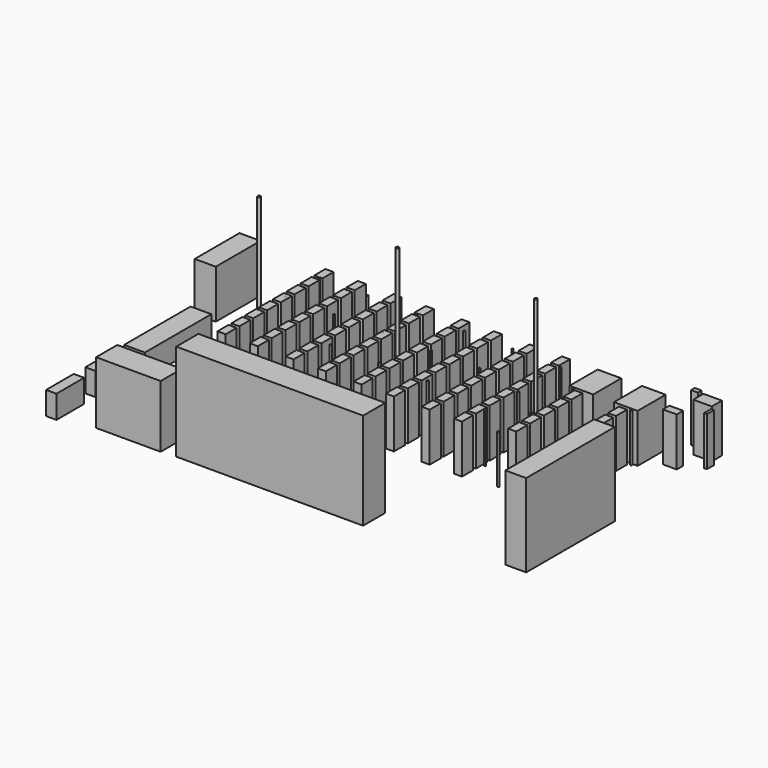
from build123d import *

# Parameters (mm, degrees)
F1_R      = 63.5
F12_DEPTH = 5486.4
F7_W      = 1041.4
F7_H      = 515.62
F13_DEPTH = 2133.6
F7_W_2    = 355.6
F7_H_2    = 609.6
F8_W      = 355.6
F8_H      = 609.6
F14_DEPTH = 2133.6
F9_W      = 355.6
F9_H      = 609.6
F15_DEPTH = 2133.6
F10_W     = 355.6
F10_H     = 609.6
F16_DEPTH = 2133.6
F11_W     = 355.6
F11_H     = 609.6
F17_DEPTH = 2133.6
F6_W      = 914.4
F6_H      = 4876.8
F18_DEPTH = 3657.6
F5_W      = 8229.6
F5_H      = 1219.2
F19_DEPTH = 4267.2
F4_W      = 1422.4
F4_H      = 1168.4
F20_DEPTH = 2743.2
F3_W      = 914.4
F3_H      = 1828.8
F21_DEPTH = 1016
F3_W_2    = 457.2
F3_H_2    = 1524
F3_H_3    = 1219.2
F2_W      = 812.8
F2_H      = 558.8
F22_DEPTH = 2133.6
F2_W_2    = 609.6
F2_H_2    = 355.6
F2_W_3    = 304.8
F2_H_3    = 203.2
F2_W_4    = 127
F2_H_4    = 406.4
F24_W     = 927.1
F24_H     = 1231.9
F25_DEPTH = 2133.6
F24_R     = 38.1


# Not quite as in the source:
# - the program builds the solid bodies; features that only make, move or delete a surface that nothing else refers to are left out


with BuildPart() as f12:
    # F1 (on face) → F12 (new body)
    with BuildSketch(Plane.XY):
        with Locations((-7657.7831685632, 0)):
            Circle(F1_R)
    extrude(amount=F12_DEPTH)


with BuildPart() as f12b:
    # F1 (on face) → F12, piece 2 (new body)
    with BuildSketch(Plane.XY):
        with Locations((-1561.7831685632, 0)):
            Circle(F1_R)
    extrude(amount=F12_DEPTH)


with BuildPart() as f12c:
    # F1 (on face) → F12, piece 3 (new body)
    with BuildSketch(Plane.XY):
        with Locations((4534.2168314368, 0)):
            Circle(F1_R)
    extrude(amount=F12_DEPTH)


with BuildPart() as f13:
    # F7 (on face) → F13 (new body)
    with BuildSketch(Plane.XY):
        with Locations((7941.9141265869, 1461.77)):
            Rectangle(F7_W, F7_H)
        with Locations((7941.9141265869, 1977.39)):
            Rectangle(F7_W, F7_H)
        with Locations((7941.9141265869, 946.15)):
            Rectangle(F7_W, F7_H)
    extrude(amount=F13_DEPTH)


with BuildPart() as f13b:
    # F7 (on face) → F13, piece 2 (new body)
    with BuildSketch(Plane.XY):
        with Locations((5986.1141265869, 1461.77)):
            Rectangle(F7_W, F7_H)
        with Locations((5986.1141265869, 1977.39)):
            Rectangle(F7_W, F7_H)
        with Locations((5986.1141265869, 946.15)):
            Rectangle(F7_W, F7_H)
    extrude(amount=F13_DEPTH)


with BuildPart() as f13c:
    # F7 (on face) → F13, piece 3 (new body)
    with BuildSketch(Plane.XY):
        with Locations((5986.1141265869, 231.14)):
            Rectangle(F7_W_2, F7_H_2)
    extrude(amount=F13_DEPTH)


with BuildPart() as f13d:
    # F7 (on face) → F13, piece 4 (new body)
    with BuildSketch(Plane.XY):
        with Locations((5986.1141265869, -530.86)):
            Rectangle(F7_W_2, F7_H_2)
    extrude(amount=F13_DEPTH)


with BuildPart() as f13e:
    # F7 (on face) → F13, piece 5 (new body)
    with BuildSketch(Plane.XY):
        with Locations((5986.1141265869, -1292.86)):
            Rectangle(F7_W_2, F7_H_2)
    extrude(amount=F13_DEPTH)


with BuildPart() as f13f:
    # F7 (on face) → F13, piece 6 (new body)
    with BuildSketch(Plane.XY):
        with Locations((7941.9141265869, 231.14)):
            Rectangle(F7_W_2, F7_H_2)
    extrude(amount=F13_DEPTH)


with BuildPart() as f13g:
    # F7 (on face) → F13, piece 7 (new body)
    with BuildSketch(Plane.XY):
        with Locations((7941.9141265869, -530.86)):
            Rectangle(F7_W_2, F7_H_2)
    extrude(amount=F13_DEPTH)


with BuildPart() as f13h:
    # F7 (on face) → F13, piece 8 (new body)
    with BuildSketch(Plane.XY):
        with Locations((7941.9141265869, -1292.86)):
            Rectangle(F7_W_2, F7_H_2)
    extrude(amount=F13_DEPTH)


with BuildPart() as f13i:
    # F7 (on face) → F13, piece 9 (new body)
    with BuildSketch(Plane.XY):
        with Locations((5986.1141265869, -2054.86)):
            Rectangle(F7_W_2, F7_H_2)
    extrude(amount=F13_DEPTH)


with BuildPart() as f13j:
    # F7 (on face) → F13, piece 10 (new body)
    with BuildSketch(Plane.XY):
        with Locations((7941.9141265869, -2054.86)):
            Rectangle(F7_W_2, F7_H_2)
    extrude(amount=F13_DEPTH)


with BuildPart() as f13k:
    # F7 (on face) → F13, piece 11 (new body)
    with BuildSketch(Plane.XY):
        with Locations((5986.1141265869, -2816.86)):
            Rectangle(F7_W_2, F7_H_2)
    extrude(amount=F13_DEPTH)


with BuildPart() as f13l:
    # F7 (on face) → F13, piece 12 (new body)
    with BuildSketch(Plane.XY):
        with Locations((7941.9141265869, -2816.86)):
            Rectangle(F7_W_2, F7_H_2)
    extrude(amount=F13_DEPTH)


with BuildPart() as f14:
    # F8 (on face) → F14 (new body)
    with BuildSketch(Plane.XY):
        with Locations((4068.4141265869, 1930.4)):
            Rectangle(F8_W, F8_H)
    extrude(amount=F14_DEPTH)


with BuildPart() as f14b:
    # F8 (on face) → F14, piece 2 (new body)
    with BuildSketch(Plane.XY):
        with Locations((4068.4141265869, 1168.4)):
            Rectangle(F8_W, F8_H)
    extrude(amount=F14_DEPTH)


with BuildPart() as f14c:
    # F8 (on face) → F14, piece 3 (new body)
    with BuildSketch(Plane.XY):
        with Locations((2646.0141265869, 1930.4)):
            Rectangle(F8_W, F8_H)
    extrude(amount=F14_DEPTH)


with BuildPart() as f14d:
    # F8 (on face) → F14, piece 4 (new body)
    with BuildSketch(Plane.XY):
        with Locations((2646.0141265869, 1168.4)):
            Rectangle(F8_W, F8_H)
    extrude(amount=F14_DEPTH)


with BuildPart() as f14e:
    # F8 (on face) → F14, piece 5 (new body)
    with BuildSketch(Plane.XY):
        with Locations((2646.0141265869, 406.4)):
            Rectangle(F8_W, F8_H)
    extrude(amount=F14_DEPTH)


with BuildPart() as f14f:
    # F8 (on face) → F14, piece 6 (new body)
    with BuildSketch(Plane.XY):
        with Locations((4068.4141265869, 406.4)):
            Rectangle(F8_W, F8_H)
    extrude(amount=F14_DEPTH)


with BuildPart() as f14g:
    # F8 (on face) → F14, piece 7 (new body)
    with BuildSketch(Plane.XY):
        with Locations((2646.0141265869, -355.6)):
            Rectangle(F8_W, F8_H)
    extrude(amount=F14_DEPTH)


with BuildPart() as f14h:
    # F8 (on face) → F14, piece 8 (new body)
    with BuildSketch(Plane.XY):
        with Locations((4068.4141265869, -355.6)):
            Rectangle(F8_W, F8_H)
    extrude(amount=F14_DEPTH)


with BuildPart() as f14i:
    # F8 (on face) → F14, piece 9 (new body)
    with BuildSketch(Plane.XY):
        with Locations((2646.0141265869, -1117.6)):
            Rectangle(F8_W, F8_H)
    extrude(amount=F14_DEPTH)


with BuildPart() as f14j:
    # F8 (on face) → F14, piece 10 (new body)
    with BuildSketch(Plane.XY):
        with Locations((4068.4141265869, -1117.6)):
            Rectangle(F8_W, F8_H)
    extrude(amount=F14_DEPTH)


with BuildPart() as f14k:
    # F8 (on face) → F14, piece 11 (new body)
    with BuildSketch(Plane.XY):
        with Locations((2646.0141265869, -1879.6)):
            Rectangle(F8_W, F8_H)
    extrude(amount=F14_DEPTH)


with BuildPart() as f14l:
    # F8 (on face) → F14, piece 12 (new body)
    with BuildSketch(Plane.XY):
        with Locations((4068.4141265869, -1879.6)):
            Rectangle(F8_W, F8_H)
    extrude(amount=F14_DEPTH)


with BuildPart() as f14m:
    # F8 (on face) → F14, piece 13 (new body)
    with BuildSketch(Plane.XY):
        with Locations((2646.014126587, -2641.6)):
            Rectangle(F8_W, F8_H)
    extrude(amount=F14_DEPTH)


with BuildPart() as f14n:
    # F8 (on face) → F14, piece 14 (new body)
    with BuildSketch(Plane.XY):
        with Locations((4068.4141265869, -2641.6)):
            Rectangle(F8_W, F8_H)
    extrude(amount=F14_DEPTH)


with BuildPart() as f14o:
    # F8 (on face) → F14, piece 15 (new body)
    with BuildSketch(Plane.XY):
        with Locations((2646.0141265869, -3403.6)):
            Rectangle(F8_W, F8_H)
    extrude(amount=F14_DEPTH)


with BuildPart() as f14p:
    # F8 (on face) → F14, piece 16 (new body)
    with BuildSketch(Plane.XY):
        with Locations((4068.4141265869, -3403.6)):
            Rectangle(F8_W, F8_H)
    extrude(amount=F14_DEPTH)


with BuildPart() as f15:
    # F9 (on face) → F15 (new body)
    with BuildSketch(Plane.XY):
        with Locations((1071.2141265869, 1930.4)):
            Rectangle(F9_W, F9_H)
    extrude(amount=F15_DEPTH)


with BuildPart() as f15b:
    # F9 (on face) → F15, piece 2 (new body)
    with BuildSketch(Plane.XY):
        with Locations((1071.2141265869, 1168.4)):
            Rectangle(F9_W, F9_H)
    extrude(amount=F15_DEPTH)


with BuildPart() as f15c:
    # F9 (on face) → F15, piece 3 (new body)
    with BuildSketch(Plane.XY):
        with Locations((-351.1858734131, 1930.4)):
            Rectangle(F9_W, F9_H)
    extrude(amount=F15_DEPTH)


with BuildPart() as f15d:
    # F9 (on face) → F15, piece 4 (new body)
    with BuildSketch(Plane.XY):
        with Locations((-351.1858734131, 1168.4)):
            Rectangle(F9_W, F9_H)
    extrude(amount=F15_DEPTH)


with BuildPart() as f15e:
    # F9 (on face) → F15, piece 5 (new body)
    with BuildSketch(Plane.XY):
        with Locations((-351.1858734131, 406.4)):
            Rectangle(F9_W, F9_H)
    extrude(amount=F15_DEPTH)


with BuildPart() as f15f:
    # F9 (on face) → F15, piece 6 (new body)
    with BuildSketch(Plane.XY):
        with Locations((1071.2141265869, 406.4)):
            Rectangle(F9_W, F9_H)
    extrude(amount=F15_DEPTH)


with BuildPart() as f15g:
    # F9 (on face) → F15, piece 7 (new body)
    with BuildSketch(Plane.XY):
        with Locations((-351.1858734131, -355.6)):
            Rectangle(F9_W, F9_H)
    extrude(amount=F15_DEPTH)


with BuildPart() as f15h:
    # F9 (on face) → F15, piece 8 (new body)
    with BuildSketch(Plane.XY):
        with Locations((1071.2141265869, -355.6)):
            Rectangle(F9_W, F9_H)
    extrude(amount=F15_DEPTH)


with BuildPart() as f15i:
    # F9 (on face) → F15, piece 9 (new body)
    with BuildSketch(Plane.XY):
        with Locations((-351.1858734131, -1117.6)):
            Rectangle(F9_W, F9_H)
    extrude(amount=F15_DEPTH)


with BuildPart() as f15j:
    # F9 (on face) → F15, piece 10 (new body)
    with BuildSketch(Plane.XY):
        with Locations((1071.2141265869, -1117.6)):
            Rectangle(F9_W, F9_H)
    extrude(amount=F15_DEPTH)


with BuildPart() as f15k:
    # F9 (on face) → F15, piece 11 (new body)
    with BuildSketch(Plane.XY):
        with Locations((-351.1858734131, -1879.6)):
            Rectangle(F9_W, F9_H)
    extrude(amount=F15_DEPTH)


with BuildPart() as f15l:
    # F9 (on face) → F15, piece 12 (new body)
    with BuildSketch(Plane.XY):
        with Locations((1071.2141265869, -1879.6)):
            Rectangle(F9_W, F9_H)
    extrude(amount=F15_DEPTH)


with BuildPart() as f15m:
    # F9 (on face) → F15, piece 13 (new body)
    with BuildSketch(Plane.XY):
        with Locations((-351.1858734131, -2641.6)):
            Rectangle(F9_W, F9_H)
    extrude(amount=F15_DEPTH)


with BuildPart() as f15n:
    # F9 (on face) → F15, piece 14 (new body)
    with BuildSketch(Plane.XY):
        with Locations((1071.2141265869, -2641.6)):
            Rectangle(F9_W, F9_H)
    extrude(amount=F15_DEPTH)


with BuildPart() as f15o:
    # F9 (on face) → F15, piece 15 (new body)
    with BuildSketch(Plane.XY):
        with Locations((-351.185873413, -3403.6)):
            Rectangle(F9_W, F9_H)
    extrude(amount=F15_DEPTH)


with BuildPart() as f15p:
    # F9 (on face) → F15, piece 16 (new body)
    with BuildSketch(Plane.XY):
        with Locations((1071.2141265869, -3403.6)):
            Rectangle(F9_W, F9_H)
    extrude(amount=F15_DEPTH)


with BuildPart() as f16:
    # F10 (on face) → F16 (new body)
    with BuildSketch(Plane.XY):
        with Locations((-1925.9858734131, 1930.4)):
            Rectangle(F10_W, F10_H)
    extrude(amount=F16_DEPTH)


with BuildPart() as f16b:
    # F10 (on face) → F16, piece 2 (new body)
    with BuildSketch(Plane.XY):
        with Locations((-1925.9858734131, 1168.4)):
            Rectangle(F10_W, F10_H)
    extrude(amount=F16_DEPTH)


with BuildPart() as f16c:
    # F10 (on face) → F16, piece 3 (new body)
    with BuildSketch(Plane.XY):
        with Locations((-3348.3858734131, 1930.4)):
            Rectangle(F10_W, F10_H)
    extrude(amount=F16_DEPTH)


with BuildPart() as f16d:
    # F10 (on face) → F16, piece 4 (new body)
    with BuildSketch(Plane.XY):
        with Locations((-3348.3858734131, 1168.4)):
            Rectangle(F10_W, F10_H)
    extrude(amount=F16_DEPTH)


with BuildPart() as f16e:
    # F10 (on face) → F16, piece 5 (new body)
    with BuildSketch(Plane.XY):
        with Locations((-3348.3858734131, 406.4)):
            Rectangle(F10_W, F10_H)
    extrude(amount=F16_DEPTH)


with BuildPart() as f16f:
    # F10 (on face) → F16, piece 6 (new body)
    with BuildSketch(Plane.XY):
        with Locations((-1925.9858734131, 406.4)):
            Rectangle(F10_W, F10_H)
    extrude(amount=F16_DEPTH)


with BuildPart() as f16g:
    # F10 (on face) → F16, piece 7 (new body)
    with BuildSketch(Plane.XY):
        with Locations((-3348.3858734131, -355.6)):
            Rectangle(F10_W, F10_H)
    extrude(amount=F16_DEPTH)


with BuildPart() as f16h:
    # F10 (on face) → F16, piece 8 (new body)
    with BuildSketch(Plane.XY):
        with Locations((-1925.9858734131, -355.6)):
            Rectangle(F10_W, F10_H)
    extrude(amount=F16_DEPTH)


with BuildPart() as f16i:
    # F10 (on face) → F16, piece 9 (new body)
    with BuildSketch(Plane.XY):
        with Locations((-3348.3858734131, -1117.6)):
            Rectangle(F10_W, F10_H)
    extrude(amount=F16_DEPTH)


with BuildPart() as f16j:
    # F10 (on face) → F16, piece 10 (new body)
    with BuildSketch(Plane.XY):
        with Locations((-1925.9858734131, -1117.6)):
            Rectangle(F10_W, F10_H)
    extrude(amount=F16_DEPTH)


with BuildPart() as f16k:
    # F10 (on face) → F16, piece 11 (new body)
    with BuildSketch(Plane.XY):
        with Locations((-3348.3858734131, -1879.6)):
            Rectangle(F10_W, F10_H)
    extrude(amount=F16_DEPTH)


with BuildPart() as f16l:
    # F10 (on face) → F16, piece 12 (new body)
    with BuildSketch(Plane.XY):
        with Locations((-1925.9858734131, -1879.6)):
            Rectangle(F10_W, F10_H)
    extrude(amount=F16_DEPTH)


with BuildPart() as f16m:
    # F10 (on face) → F16, piece 13 (new body)
    with BuildSketch(Plane.XY):
        with Locations((-3348.3858734131, -2641.6)):
            Rectangle(F10_W, F10_H)
    extrude(amount=F16_DEPTH)


with BuildPart() as f16n:
    # F10 (on face) → F16, piece 14 (new body)
    with BuildSketch(Plane.XY):
        with Locations((-1925.9858734131, -2641.6)):
            Rectangle(F10_W, F10_H)
    extrude(amount=F16_DEPTH)


with BuildPart() as f16o:
    # F10 (on face) → F16, piece 15 (new body)
    with BuildSketch(Plane.XY):
        with Locations((-3348.385873413, -3403.6)):
            Rectangle(F10_W, F10_H)
    extrude(amount=F16_DEPTH)


with BuildPart() as f16p:
    # F10 (on face) → F16, piece 16 (new body)
    with BuildSketch(Plane.XY):
        with Locations((-1925.9858734131, -3403.6)):
            Rectangle(F10_W, F10_H)
    extrude(amount=F16_DEPTH)


with BuildPart() as f17:
    # F11 (on face) → F17 (new body)
    with BuildSketch(Plane.XY):
        with Locations((-4923.1858734131, 1930.4)):
            Rectangle(F11_W, F11_H)
    extrude(amount=F17_DEPTH)


with BuildPart() as f17b:
    # F11 (on face) → F17, piece 2 (new body)
    with BuildSketch(Plane.XY):
        with Locations((-4923.1858734131, 1168.4)):
            Rectangle(F11_W, F11_H)
    extrude(amount=F17_DEPTH)


with BuildPart() as f17c:
    # F11 (on face) → F17, piece 3 (new body)
    with BuildSketch(Plane.XY):
        with Locations((-6345.5858734131, 1930.4)):
            Rectangle(F11_W, F11_H)
    extrude(amount=F17_DEPTH)


with BuildPart() as f17d:
    # F11 (on face) → F17, piece 4 (new body)
    with BuildSketch(Plane.XY):
        with Locations((-6345.5858734131, 1168.4)):
            Rectangle(F11_W, F11_H)
    extrude(amount=F17_DEPTH)


with BuildPart() as f17e:
    # F11 (on face) → F17, piece 5 (new body)
    with BuildSketch(Plane.XY):
        with Locations((-6345.5858734131, 406.4)):
            Rectangle(F11_W, F11_H)
    extrude(amount=F17_DEPTH)


with BuildPart() as f17f:
    # F11 (on face) → F17, piece 6 (new body)
    with BuildSketch(Plane.XY):
        with Locations((-4923.1858734131, 406.4)):
            Rectangle(F11_W, F11_H)
    extrude(amount=F17_DEPTH)


with BuildPart() as f17g:
    # F11 (on face) → F17, piece 7 (new body)
    with BuildSketch(Plane.XY):
        with Locations((-4923.1858734131, -355.6)):
            Rectangle(F11_W, F11_H)
    extrude(amount=F17_DEPTH)


with BuildPart() as f17h:
    # F11 (on face) → F17, piece 8 (new body)
    with BuildSketch(Plane.XY):
        with Locations((-4923.1858734131, -1117.6)):
            Rectangle(F11_W, F11_H)
    extrude(amount=F17_DEPTH)


with BuildPart() as f17i:
    # F11 (on face) → F17, piece 9 (new body)
    with BuildSketch(Plane.XY):
        with Locations((-4923.1858734131, -1879.6)):
            Rectangle(F11_W, F11_H)
    extrude(amount=F17_DEPTH)


with BuildPart() as f17j:
    # F11 (on face) → F17, piece 10 (new body)
    with BuildSketch(Plane.XY):
        with Locations((-4923.1858734131, -2641.6)):
            Rectangle(F11_W, F11_H)
    extrude(amount=F17_DEPTH)


with BuildPart() as f17k:
    # F11 (on face) → F17, piece 11 (new body)
    with BuildSketch(Plane.XY):
        with Locations((-4923.1858734131, -3403.6)):
            Rectangle(F11_W, F11_H)
    extrude(amount=F17_DEPTH)


with BuildPart() as f17l:
    # F11 (on face) → F17, piece 12 (new body)
    with BuildSketch(Plane.XY):
        with Locations((-6345.5858734131, -355.6)):
            Rectangle(F11_W, F11_H)
    extrude(amount=F17_DEPTH)


with BuildPart() as f17m:
    # F11 (on face) → F17, piece 13 (new body)
    with BuildSketch(Plane.XY):
        with Locations((-6345.5858734131, -1117.6)):
            Rectangle(F11_W, F11_H)
    extrude(amount=F17_DEPTH)


with BuildPart() as f17n:
    # F11 (on face) → F17, piece 14 (new body)
    with BuildSketch(Plane.XY):
        with Locations((-6345.5858734131, -1879.6)):
            Rectangle(F11_W, F11_H)
    extrude(amount=F17_DEPTH)


with BuildPart() as f17o:
    # F11 (on face) → F17, piece 15 (new body)
    with BuildSketch(Plane.XY):
        with Locations((-6345.5858734131, -2641.6)):
            Rectangle(F11_W, F11_H)
    extrude(amount=F17_DEPTH)


with BuildPart() as f17p:
    # F11 (on face) → F17, piece 16 (new body)
    with BuildSketch(Plane.XY):
        with Locations((-6345.5858734131, -3403.6)):
            Rectangle(F11_W, F11_H)
    extrude(amount=F17_DEPTH)


with BuildPart() as f18:
    # F6 (on face) → F18 (new body)
    with BuildSketch(Plane.XY):
        with Locations((9969.8168314368, -5461)):
            Rectangle(F6_W, F6_H)
    extrude(amount=F18_DEPTH)


with BuildPart() as f19:
    # F5 (on face) → F19 (new body)
    with BuildSketch(Plane.XY):
        with Locations((-240.9831685632, -8077.2)):
            Rectangle(F5_W, F5_H)
    extrude(amount=F19_DEPTH)


with BuildPart() as f20:
    # F4 (on face) → F20 (new body)
    with BuildSketch(Plane.XY):
        with Locations((-7135.7371807098, -8153.4)):
            Rectangle(F4_W, F4_H)
        with Locations((-5713.3371807098, -8153.4)):
            Rectangle(F4_W, F4_H)
    extrude(amount=F20_DEPTH)


with BuildPart() as f21:
    # F3 (on face) → F21 (new body)
    with BuildSketch(Plane.XY):
        with Locations((-9283.3831685632, -2082.8)):
            Rectangle(F3_W, F3_H)
        with Locations((-9283.3831685632, -3911.6)):
            Rectangle(F3_W, F3_H)
    extrude(amount=F21_DEPTH)


with BuildPart() as f21b:
    # F3 (on face) → F21, piece 2 (new body)
    with BuildSketch(Plane.XY):
        with Locations((-9511.9831685632, -8360.1227645874)):
            Rectangle(F3_W_2, F3_H_2)
    extrude(amount=F21_DEPTH)


with BuildPart() as f21c:
    # F3 (on face) → F21, piece 3 (new body)
    with BuildSketch(Plane.XY):
        with Locations((-9511.9831685632, -6350)):
            Rectangle(F3_W_2, F3_H_3)
    extrude(amount=F21_DEPTH)


with BuildPart() as f22:
    # F2 (on face) → F22 (new body)
    with BuildSketch(Plane.XY):
        with Locations((9842.8168314368, 2819.4)):
            Rectangle(F2_W, F2_H)
    extrude(amount=F22_DEPTH)


with BuildPart() as f22b:
    # F2 (on face) → F22, piece 2 (new body)
    with BuildSketch(Plane.XY):
        with Locations((9377.0141265869, 1498.6)):
            Rectangle(F2_W_2, F2_H_2)
    extrude(amount=F22_DEPTH)


with BuildPart() as f22c:
    # F2 (on face) → F22, piece 3 (new body)
    with BuildSketch(Plane.XY):
        with Locations((9080.8168314368, 3149.6)):
            Rectangle(F2_W_3, F2_H_3)
    extrude(amount=F22_DEPTH)


with BuildPart() as f22d:
    # F2 (on face) → F22, piece 4 (new body)
    with BuildSketch(Plane.XY):
        with Locations((10414.3168314368, 2184.4)):
            Rectangle(F2_W_4, F2_H_4)
    extrude(amount=F22_DEPTH)


with BuildPart() as f25:
    # F24 (on face) → F25 (new body)
    with BuildSketch(Plane.XY):
        with Locations((-10037.7631685632, 628.65)):
            Rectangle(F24_W, F24_H)
        with Locations((-10037.7631685632, 1860.55)):
            Rectangle(F24_W, F24_H)
    extrude(amount=F25_DEPTH)


with BuildPart() as f25b:
    # F24 (on face) → F25, piece 2 (new body)
    with BuildSketch(Plane.XY):
        with Locations((-6307.4858734131, 1603.375)):
            Circle(F24_R)
    extrude(amount=F25_DEPTH)


with BuildPart() as f25c:
    # F24 (on face) → F25, piece 3 (new body)
    with BuildSketch(Plane.XY):
        with Locations((-6307.4858734131, -225.425)):
            Circle(F24_R)
    extrude(amount=F25_DEPTH)


with BuildPart() as f25d:
    # F24 (on face) → F25, piece 4 (new body)
    with BuildSketch(Plane.XY):
        with Locations((-4173.8858734131, 1603.375)):
            Circle(F24_R)
    extrude(amount=F25_DEPTH)


with BuildPart() as f25e:
    # F24 (on face) → F25, piece 5 (new body)
    with BuildSketch(Plane.XY):
        with Locations((-4173.8858734131, -225.425)):
            Circle(F24_R)
    extrude(amount=F25_DEPTH)


with BuildPart() as f25f:
    # F24 (on face) → F25, piece 6 (new body)
    with BuildSketch(Plane.XY):
        with Locations((-2040.2858734131, -225.425)):
            Circle(F24_R)
    extrude(amount=F25_DEPTH)


with BuildPart() as f25g:
    # F24 (on face) → F25, piece 7 (new body)
    with BuildSketch(Plane.XY):
        with Locations((-2040.2858734131, 1603.375)):
            Circle(F24_R)
    extrude(amount=F25_DEPTH)


with BuildPart() as f25h:
    # F24 (on face) → F25, piece 8 (new body)
    with BuildSketch(Plane.XY):
        with Locations((93.3141265869, 1603.375)):
            Circle(F24_R)
    extrude(amount=F25_DEPTH)


with BuildPart() as f25i:
    # F24 (on face) → F25, piece 9 (new body)
    with BuildSketch(Plane.XY):
        with Locations((93.3141265869, -225.425)):
            Circle(F24_R)
    extrude(amount=F25_DEPTH)


with BuildPart() as f25j:
    # F24 (on face) → F25, piece 10 (new body)
    with BuildSketch(Plane.XY):
        with Locations((2226.9141265869, 1603.375)):
            Circle(F24_R)
    extrude(amount=F25_DEPTH)


with BuildPart() as f25k:
    # F24 (on face) → F25, piece 11 (new body)
    with BuildSketch(Plane.XY):
        with Locations((2226.9141265869, -225.425)):
            Circle(F24_R)
    extrude(amount=F25_DEPTH)


with BuildPart() as f25l:
    # F24 (on face) → F25, piece 12 (new body)
    with BuildSketch(Plane.XY):
        with Locations((5681.3141265869, 612.14)):
            Circle(F24_R)
    extrude(amount=F25_DEPTH)


with BuildPart() as f25m:
    # F24 (on face) → F25, piece 13 (new body)
    with BuildSketch(Plane.XY):
        with Locations((4360.5141265869, 1574.8)):
            Circle(F24_R)
    extrude(amount=F25_DEPTH)


with BuildPart() as f25n:
    # F24 (on face) → F25, piece 14 (new body)
    with BuildSketch(Plane.XY):
        with Locations((8246.7141265869, 612.14)):
            Circle(F24_R)
    extrude(amount=F25_DEPTH)


with BuildPart() as f25o:
    # F24 (on face) → F25, piece 15 (new body)
    with BuildSketch(Plane.XY):
        with Locations((4360.5141265869, -749.3)):
            Circle(F24_R)
    extrude(amount=F25_DEPTH)


with BuildPart() as f25p:
    # F24 (on face) → F25, piece 16 (new body)
    with BuildSketch(Plane.XY):
        with Locations((5681.3141265869, -1673.86)):
            Circle(F24_R)
    extrude(amount=F25_DEPTH)


with BuildPart() as f25q:
    # F24 (on face) → F25, piece 17 (new body)
    with BuildSketch(Plane.XY):
        with Locations((8246.7141265869, -1673.86)):
            Circle(F24_R)
    extrude(amount=F25_DEPTH)


with BuildPart() as f25r:
    # F24 (on face) → F25, piece 18 (new body)
    with BuildSketch(Plane.XY):
        with Locations((8246.7141265869, -3502.66)):
            Circle(F24_R)
    extrude(amount=F25_DEPTH)


with BuildPart() as f25s:
    # F24 (on face) → F25, piece 19 (new body)
    with BuildSketch(Plane.XY):
        with Locations((5681.3141265869, -3502.66)):
            Circle(F24_R)
    extrude(amount=F25_DEPTH)


with BuildPart() as f25t:
    # F24 (on face) → F25, piece 20 (new body)
    with BuildSketch(Plane.XY):
        with Locations((4360.5141265869, -2578.1)):
            Circle(F24_R)
    extrude(amount=F25_DEPTH)


with BuildPart() as f25u:
    # F24 (on face) → F25, piece 21 (new body)
    with BuildSketch(Plane.XY):
        with Locations((1414.1141265869, -2054.225)):
            Circle(F24_R)
    extrude(amount=F25_DEPTH)


with BuildPart() as f25v:
    # F24 (on face) → F25, piece 22 (new body)
    with BuildSketch(Plane.XY):
        with Locations((-719.4858734131, -2054.225)):
            Circle(F24_R)
    extrude(amount=F25_DEPTH)


with BuildPart() as f25w:
    # F24 (on face) → F25, piece 23 (new body)
    with BuildSketch(Plane.XY):
        with Locations((-2853.0858734131, -2054.225)):
            Circle(F24_R)
    extrude(amount=F25_DEPTH)


solid = Compound([f12.part, f12b.part, f12c.part, f13.part, f13b.part, f13c.part, f13d.part, f13e.part, f13f.part, f13g.part, f13h.part, f13i.part, f13j.part, f13k.part, f13l.part, f14.part, f14b.part, f14c.part, f14d.part, f14e.part, f14f.part, f14g.part, f14h.part, f14i.part, f14j.part, f14k.part, f14l.part, f14m.part, f14n.part, f14o.part, f14p.part, f15.part, f15b.part, f15c.part, f15d.part, f15e.part, f15f.part, f15g.part, f15h.part, f15i.part, f15j.part, f15k.part, f15l.part, f15m.part, f15n.part, f15o.part, f15p.part, f16.part, f16b.part, f16c.part, f16d.part, f16e.part, f16f.part, f16g.part, f16h.part, f16i.part, f16j.part, f16k.part, f16l.part, f16m.part, f16n.part, f16o.part, f16p.part, f17.part, f17b.part, f17c.part, f17d.part, f17e.part, f17f.part, f17g.part, f17h.part, f17i.part, f17j.part, f17k.part, f17l.part, f17m.part, f17n.part, f17o.part, f17p.part, f18.part, f19.part, f20.part, f21.part, f21b.part, f21c.part, f22.part, f22b.part, f22c.part, f22d.part, f25.part, f25b.part, f25c.part, f25d.part, f25e.part, f25f.part, f25g.part, f25h.part, f25i.part, f25j.part, f25k.part, f25l.part, f25m.part, f25n.part, f25o.part, f25p.part, f25q.part, f25r.part, f25s.part, f25t.part, f25u.part, f25v.part, f25w.part])
